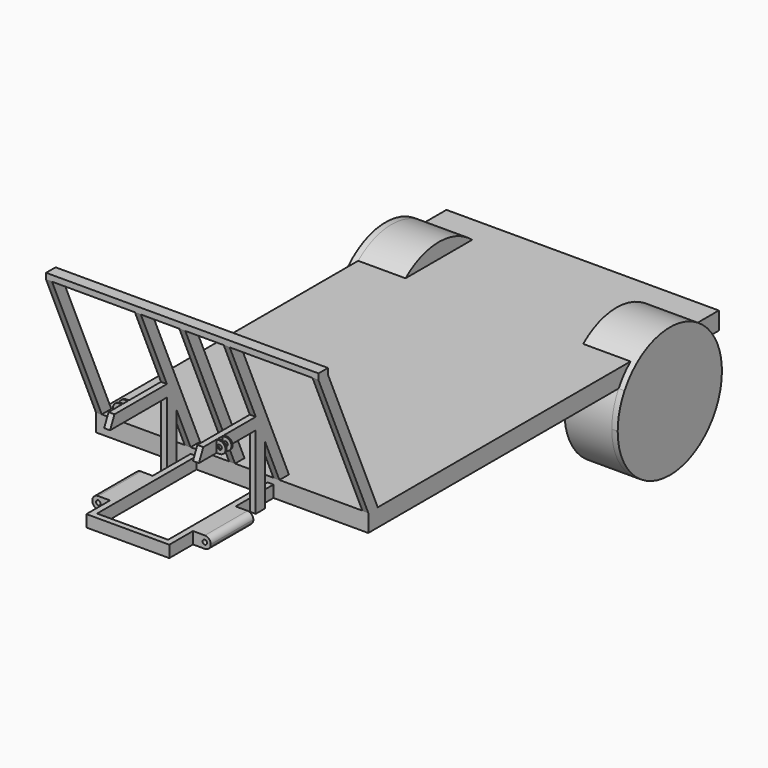
from build123d import *

# Parameters (mm, degrees)
F0_W           = 1168.4
F0_H           = 1879.6
F1_DEPTH       = 76.2
F2_R           = 279.4
F3_DEPTH       = 203.2
F3_DEPTH_BACK  = 25.4
F5_DEPTH       = 203.2
F5_DEPTH_BACK  = 25.4
F6_W           = 25.4
F6_H           = 558.8
F7_DEPTH       = 50.8
F9_DEPTH       = 25.4
F11_DEPTH      = 25.4
F12_W          = 50.8
F12_H          = 25.4
F13_DEPTH      = 1168.4
F17_DEPTH      = 12.7
F17_DEPTH_BACK = 12.7
F18_W          = 228.6
F18_H          = 50.8
F19_DEPTH      = 76.2
F20_R          = 9.525
F21_DEPTH      = 228.6
F23_DEPTH      = 25.4
F24_W          = 6.35
F24_H          = 50.8
F25_DEPTH      = 38.1
F26_R          = 9.525
F27_DEPTH      = 50.8
F29_W          = 25.4
F29_H          = 50.8
F30_DEPTH      = 304.8


with BuildPart() as f1:
    # F0 (on Top) → F1 (new body)
    with BuildSketch(Plane.XY):
        with Locations((584.2, 939.8)):
            Rectangle(F0_W, F0_H)
    extrude(amount=F1_DEPTH)

    # F2 (on face) → F3 (join, two sides)
    with BuildSketch(Plane(origin=(0, 0, 0), x_dir=(0, -1, 0), z_dir=(-1, 0, 0))) as f3_sk:
        with Locations((-1585.070014, -138.537094)):
            Circle(F2_R)
    extrude(amount=-F3_DEPTH)
    extrude(f3_sk.sketch, amount=F3_DEPTH_BACK)

    # F4 (on face) → F5 (join, two sides)
    with BuildSketch(Plane.YZ.offset(1168.4)) as f5_sk:
        with BuildLine():
            ThreePointArc((1864.470014, -138.537094), (1855.122445, -66.870892), (1827.7052, 0))
            Line((1827.7052, 0), (1342.434828, 0))
            ThreePointArc((1342.434828, 0), (1513.403812, -408.589525), (1864.470014, -138.537094))
        make_face()
        with BuildLine():
            Line((1342.434828, 0), (1827.7052, 0))
            ThreePointArc((1827.7052, 0), (1585.070014, 140.862906), (1342.434828, 0))
        make_face()
    extrude(amount=-F5_DEPTH)
    extrude(f5_sk.sketch, amount=F5_DEPTH_BACK)

    # F6 (on face) → F7 (join)
    with BuildSketch(Plane(origin=(0, 0, 0), x_dir=(1, 0, 0), z_dir=(0, 0, -1))):
        with Locations((419.1, 279.4)):
            Rectangle(F6_W, F6_H)
        with Locations((749.3, 279.4)):
            Rectangle(F6_W, F6_H)
    extrude(amount=-F7_DEPTH)

    # F8 (on face) → F9 (join)
    with BuildSketch(Plane(origin=(0, 0, 0), x_dir=(0, -1, 0), z_dir=(-1, 0, 0))):
        Polygon((216.077259, 685.8), (-50.8, 76.2), (0, 76.2), (266.877259, 685.8), align=None)
    extrude(amount=-F9_DEPTH)

    # F10 (on face) → F11 (join)
    with BuildSketch(Plane.YZ.offset(1168.4)):
        Polygon((-216.077259, 685.8), (-266.877259, 685.8), (0, 76.2), (50.8, 76.2), align=None)
    extrude(amount=-F11_DEPTH)

    # F12 (on face) → F13 (join, through all)
    with BuildSketch(Plane.YZ.offset(1168.4)):
        with Locations((-241.477259, 698.5)):
            Rectangle(F12_W, F12_H)
    extrude(amount=-F13_DEPTH)

    # F16 (on line) → F17 (join, two sides)
    with BuildSketch(Plane(origin=(584.2, 0, 0), x_dir=(0, -1, 0), z_dir=(-1, 0, 0))) as f17_sk:
        Polygon((216.077259, 685.8), (-50.8, 76.2), (0, 76.2), (266.877259, 685.8), align=None)
    extrude(amount=F17_DEPTH)
    extrude(f17_sk.sketch, amount=-F17_DEPTH_BACK)

    # F18 (on face) → F19 (join)
    with BuildSketch(Plane(origin=(406.4, 0, 0), x_dir=(0, -1, 0), z_dir=(-1, 0, 0))):
        with Locations((317.5, 25.4)):
            Rectangle(F18_W, F18_H)
    extrude(amount=F19_DEPTH)

    # F20 (on face) → F21 (cut, through all)
    with BuildSketch(Plane.XZ.offset(431.8)):
        with BuildLine():
            ThreePointArc((330.2, 25.4), (337.639488, 43.360512), (355.6, 50.8))
            Line((355.6, 50.8), (330.2, 50.8))
            Line((330.2, 50.8), (330.2, 25.4))
        make_face()
        with Locations((355.6, 25.4)):
            Circle(F20_R)
        with BuildLine():
            Line((330.2, 0), (355.6, 0))
            ThreePointArc((355.6, 0), (337.639488, 7.439488), (330.2, 25.4))
            Line((330.2, 25.4), (330.2, 0))
        make_face()
    extrude(amount=-F21_DEPTH, mode=Mode.SUBTRACT)

    # F22 (on face) → F23 (join)
    with BuildSketch(Plane(origin=(406.4, 0, 0), x_dir=(0, -1, 0), z_dir=(-1, 0, 0))):
        Polygon((266.877259, 685.8), (216.077259, 685.8), (127, 482.33007), (127, 366.292907), align=None)
        Polygon((127, 366.292907), (127, 482.33007), (76.2, 366.292907), align=None)
        Polygon((76.2, 315.492907), (76.2, 366.292907), (53.960228, 315.492907), align=None)
        Polygon((127, 366.292907), (76.2, 366.292907), (76.2, 315.492907), (104.760228, 315.492907), align=None)
        Polygon((127, 315.492907), (127, 366.292907), (104.760228, 315.492907), align=None)
        Polygon((408.111571, 366.292907), (127, 366.292907), (127, 315.492907), (431.8, 315.492907), align=None)
        Polygon((76.2, 315.492907), (53.960228, 315.492907), (-50.8, 76.2), (0, 76.2), (76.2, 250.255744), align=None)
        Polygon((104.760228, 315.492907), (76.2, 315.492907), (76.2, 250.255744), align=None)
        Polygon((127, 315.492907), (104.760228, 315.492907), (76.2, 250.255744), (76.2, 0), (127, 0), align=None)
    extrude(amount=F23_DEPTH)

    # F24 (on face) → F25 (join)
    with BuildSketch(Plane(origin=(381, 0, 0), x_dir=(0, -1, 0), z_dir=(-1, 0, 0))):
        with Locations((301.625, 340.892907)):
            Rectangle(F24_W, F24_H)
        with Locations((333.375, 340.892907)):
            Rectangle(F24_W, F24_H)
    extrude(amount=F25_DEPTH)

    # F26 (on face) → F27 (cut)
    with BuildSketch(Plane.XZ.offset(336.55)):
        with BuildLine():
            ThreePointArc((342.9, 340.892907), (350.339488, 358.853419), (368.3, 366.292907))
            Line((368.3, 366.292907), (342.9, 366.292907))
            Line((342.9, 366.292907), (342.9, 340.892907))
        make_face()
        with Locations((368.3, 340.892907)):
            Circle(F26_R)
        with BuildLine():
            Line((342.9, 315.492907), (368.3, 315.492907))
            ThreePointArc((368.3, 315.492907), (350.339488, 322.932395), (342.9, 340.892907))
            Line((342.9, 340.892907), (342.9, 315.492907))
        make_face()
    extrude(amount=-F27_DEPTH, mode=Mode.SUBTRACT)

    # F28: F1 across plane


with BuildPart() as f1_1:
    add(f1.part)
    add(f1.part.mirror(Plane(origin=(584.2, 0, 0), x_dir=(0, -1, 0), z_dir=(-1, 0, 0))))

    # F29 (on face) → F30 (join, through all)
    with BuildSketch(Plane(origin=(736.6, 0, 0), x_dir=(0, -1, 0), z_dir=(-1, 0, 0))):
        with Locations((546.1, 25.4)):
            Rectangle(F29_W, F29_H)
    extrude(amount=F30_DEPTH)


solid = f1_1.part
